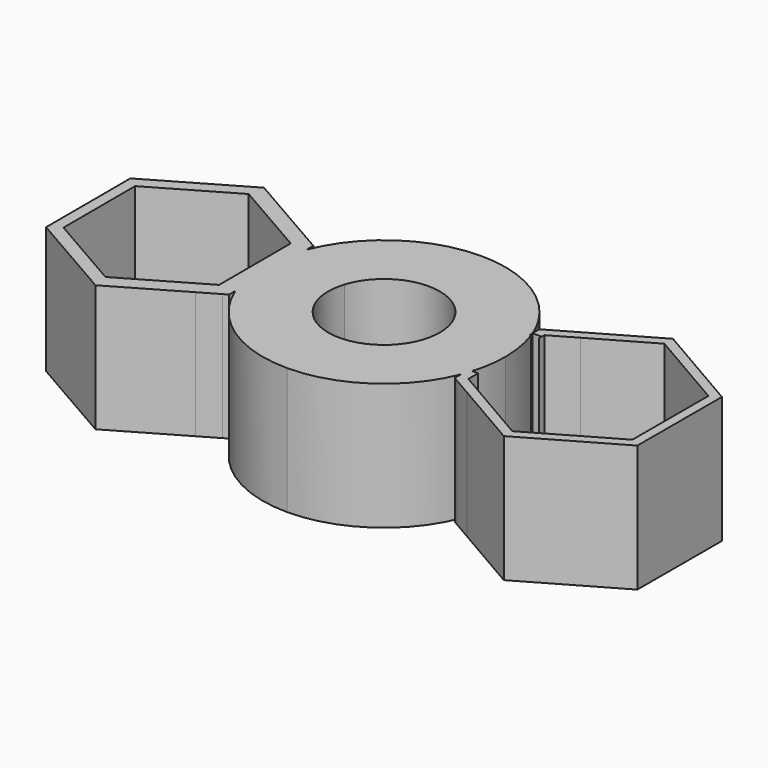
from build123d import *

# Parameters (mm, degrees)
F1_DEPTH = 25
F3_DEPTH = 25


with BuildPart() as f1:
    # F0 (on Top) → F1 (new body)
    with BuildSketch(Plane.XY):
        with BuildLine():
            ThreePointArc((-10.4646871668, 3.3897378218), (1.7158731254, 10.8653476437), (11, 0))
            ThreePointArc((11, 0), (10.8653476437, -1.7158731254), (10.4646871668, -3.3897378218))
            ThreePointArc((10.4646871668, -3.3897378218), (11.5303364364, -16.8717211773), (0, -23.9393109523))
            ThreePointArc((0, -23.9393109523), (13.4535838876, -19.8013052461), (22.2561561395, -8.8178298218))
            Line((22.2561561395, -8.8178298218), (22.2834265087, 8.7486862959))
            ThreePointArc((22.2834265087, 8.7486862959), (21.5168684816, 10.4935684883), (20.6139374132, 12.1719428685))
            Line((20.6139374132, 12.1719428685), (20.4327683896, 12.1719428685))
            Line((20.4327683896, 12.1719428685), (20.4327683896, 12.4736756736))
            ThreePointArc((20.4327683896, 12.4736756736), (11.7149350874, 20.8770425293), (0, 23.9393109523))
            ThreePointArc((0, 23.9393109523), (-11.5303364364, 16.8717211773), (-10.4646871668, 3.3897378218))
        make_face()
        with BuildLine():
            ThreePointArc((10.4646871668, -3.3897378218), (-3.3897378218, -10.4646871668), (-10.4646871668, 3.3897378218))
            ThreePointArc((-10.4646871668, 3.3897378218), (-11.5303364364, 16.8717211773), (0, 23.9393109523))
            ThreePointArc((0, 23.9393109523), (-13.4843073091, 19.7803959836), (-22.2834265087, 8.7486862959))
            Line((-22.2834265087, 8.7486862959), (-22.2561561395, -8.8178298218))
            ThreePointArc((-22.2561561395, -8.8178298218), (-13.4535838876, -19.8013052461), (0, -23.9393109523))
            ThreePointArc((0, -23.9393109523), (11.5303364364, -16.8717211773), (10.4646871668, -3.3897378218))
        make_face()
        with BuildLine():
            ThreePointArc((20.6139374132, 12.1719428685), (20.5239074006, 12.3231422082), (20.4327683896, 12.4736756736))
            Line((20.4327683896, 12.4736756736), (20.4327683896, 12.1719428685))
            Line((20.4327683896, 12.1719428685), (20.6139374132, 12.1719428685))
        make_face()
        with BuildLine():
            Line((-22.2561561395, -8.8178298218), (-22.2834265087, 8.7486862959))
            ThreePointArc((-22.2834265087, 8.7486862959), (-22.3171762669, 8.6622313721), (-22.3505905999, 8.5756462558))
            ThreePointArc((-22.3505905999, 8.5756462558), (-22.9180889493, 6.917500111), (-23.3627568452, 5.2222793359))
            ThreePointArc((-23.3627568452, 5.2222793359), (-23.9236754966, -0.865077803), (-22.9245601537, -6.8960242628))
            ThreePointArc((-22.9245601537, -6.8960242628), (-22.876956445, -7.0523381007), (-22.8282869054, -7.2083233721))
            ThreePointArc((-22.8282869054, -7.2083233721), (-22.5565817206, -8.0181812122), (-22.2561561395, -8.8178298218))
        make_face()
        with BuildLine():
            ThreePointArc((-22.3505905999, 8.5756462558), (-22.3171762669, 8.6622313721), (-22.2834265087, 8.7486862959))
            Line((-22.2834265087, 8.7486862959), (-22.2860376354, 10.4306730632))
            Line((-22.2860376354, 10.4306730632), (-26.9655953528, 13.1227395452))
            Line((-26.9655953528, 13.1227395452), (-28.876762415, 14.2222000286))
            Line((-28.876762415, 14.2222000286), (-40.3201948997, 20.8054035902))
            Line((-40.3201948997, 20.8054035902), (-58.3220537256, 10.374730527))
            Line((-58.3220537256, 10.374730527), (-58.2897552873, -10.4306730632))
            Line((-58.2897552873, -10.4306730632), (-40.2555980231, -20.8054035902))
            Line((-40.2555980231, -20.8054035902), (-26.7618837097, -12.9868486414))
            Line((-26.7618837097, -12.9868486414), (-23.1227707365, -10.8782665205))
            Line((-23.1227707365, -10.8782665205), (-22.2537391971, -10.374730527))
            Line((-22.2537391971, -10.374730527), (-22.2561561395, -8.8178298218))
            ThreePointArc((-22.2561561395, -8.8178298218), (-22.5565817206, -8.0181812122), (-22.8282869054, -7.2083233721))
            ThreePointArc((-22.8282869054, -7.2083233721), (-22.876956445, -7.0523381007), (-22.9245601537, -6.8960242628))
            ThreePointArc((-22.9245601537, -6.8960242628), (-23.9236754966, -0.865077803), (-23.3627568452, 5.2222793359))
            ThreePointArc((-23.3627568452, 5.2222793359), (-22.9180889493, 6.917500111), (-22.3505905999, 8.5756462558))
        make_face()
        with BuildLine():
            Line((22.2834265087, 8.7486862959), (22.2561561395, -8.8178298218))
            ThreePointArc((22.2561561395, -8.8178298218), (22.6061950021, -7.8772175544), (22.9165006409, -6.9227600889))
            Line((22.9165006409, -6.9227600889), (22.9165006409, -6.5203195466))
            Line((22.9165006409, -6.5203195466), (23.0342362991, -6.5203195466))
            ThreePointArc((23.0342362991, -6.5203195466), (23.7119627423, -3.291417898), (23.9393109523, 0))
            ThreePointArc((23.9393109523, 0), (23.5915816395, 4.0654501127), (22.5584955519, 8.0127952242))
            Line((22.5584955519, 8.0127952242), (22.2926987152, 8.0127952242))
            Line((22.2926987152, 8.0127952242), (22.2926987152, 8.7250325423))
            ThreePointArc((22.2926987152, 8.7250325423), (22.2880657498, 8.7368606491), (22.2834265087, 8.7486862959))
        make_face()
        with BuildLine():
            ThreePointArc((22.9165006409, -6.9227600889), (22.6061950021, -7.8772175544), (22.2561561395, -8.8178298218))
            Line((22.2561561395, -8.8178298218), (22.2537391971, -10.374730527))
            Line((22.2537391971, -10.374730527), (23.1227707365, -10.8782665205))
            Line((23.1227707365, -10.8782665205), (26.7618837097, -12.9868486414))
            Line((26.7618837097, -12.9868486414), (40.2555980231, -20.8054035902))
            Line((40.2555980231, -20.8054035902), (58.2897552873, -10.4306730632))
            Line((58.2897552873, -10.4306730632), (58.3220537256, 10.374730527))
            Line((58.3220537256, 10.374730527), (40.3201948997, 20.8054035902))
            Line((40.3201948997, 20.8054035902), (28.876762415, 14.2222000286))
            Line((28.876762415, 14.2222000286), (28.9680806238, 14.2222000286))
            Line((28.9680806238, 14.2222000286), (28.9680806238, 12.1719428685))
            Line((28.9680806238, 12.1719428685), (40.3201948997, 18.6999721072))
            Line((40.3201948997, 18.6999721072), (56.4986965755, 9.3220147855))
            Line((56.4986965755, 9.3220147855), (56.4663981371, -9.3779573217))
            Line((56.4663981371, -9.3779573217), (40.2555980231, -18.6999721072))
            Line((40.2555980231, -18.6999721072), (24.0770963473, -9.3220147855))
            Line((24.0770963473, -9.3220147855), (24.0812403203, -6.9227600889))
            Line((24.0812403203, -6.9227600889), (22.9165006409, -6.9227600889))
        make_face()
        with BuildLine():
            Line((22.2860376354, 10.4306730632), (22.2834265087, 8.7486862959))
            ThreePointArc((22.2834265087, 8.7486862959), (22.2880657498, 8.7368606491), (22.2926987152, 8.7250325423))
            Line((22.2926987152, 8.7250325423), (24.1070368889, 8.7250325423))
            Line((24.1070368889, 8.7250325423), (24.1070368889, 8.0127952242))
            Line((24.1070368889, 8.0127952242), (24.1093947856, 9.3779573217))
            Line((24.1093947856, 9.3779573217), (28.9680806238, 12.1719428685))
            Line((28.9680806238, 12.1719428685), (28.9680806238, 14.2222000286))
            Line((28.9680806238, 14.2222000286), (28.876762415, 14.2222000286))
            Line((28.876762415, 14.2222000286), (26.9655953528, 13.1227395452))
            Line((26.9655953528, 13.1227395452), (22.2860376354, 10.4306730632))
        make_face()
    extrude(amount=F1_DEPTH)

    # F2 (on face) → F3 (cut)
    with BuildSketch(Plane.XY.offset(25)):
        Polygon((-56.1096642619, -8.8687674562), (-40.7759704459, -17.6899693007), (-25.4697386486, -8.8212018445), (-25.4972006673, 8.8687674562), (-40.8308944833, 17.6899693007), (-56.1371262806, 8.8212018445), align=None)
    extrude(amount=-F3_DEPTH, mode=Mode.SUBTRACT)


solid = f1.part
